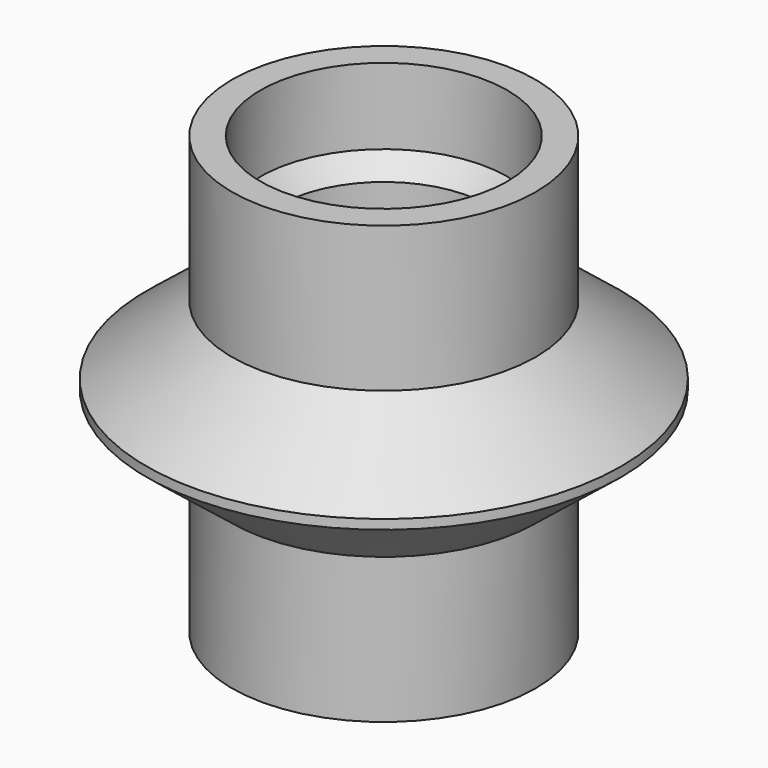
from build123d import *

# Parameters (mm, degrees)
F0_R         = 8
F0_R_2       = 6.5
F1_DEPTH     = 11.5
F0_R_3       = 12.5
F2_DEPTH     = 4.25
F3_S5_R      = 8
F3_T6_DEPTH  = 19
F3_S11_R     = 8
F3_T12_DEPTH = 19
F0_R_4       = 5.5
F5_DEPTH     = 7.5
F6_SIZE      = 0.99999


# Not quite as in the source:
# - a fillet or chamfer that OpenCascade refuses, or shapes differently, is made with other operations: its cross-section is extruded or revolved along the edge and cut away or added
# - two fillets or chamfers of one size are made in one step
# - a fillet or chamfer is up to 0.001 mm smaller than in the source, because OpenCascade refuses the exact size


with BuildPart() as f1:
    # F0 (on Top) → F1 (new body, symmetric)
    with BuildSketch(Plane.XY):
        Circle(F0_R)
        Circle(F0_R_2, mode=Mode.SUBTRACT)
    extrude(amount=F1_DEPTH, both=True)

    # F0 (on Top) → F2 (join, symmetric)
    with BuildSketch(Plane.XY):
        Circle(F0_R_3)
        Circle(F0_R, mode=Mode.SUBTRACT)
    extrude(amount=F2_DEPTH, both=True)

    # F3: chamfer of 5 x 4 on 2 edges, made by hand


with BuildPart() as f3_tool2:
    # F3_s3 → F3_t4 (revolve)
    with BuildSketch(Plane.XZ):
        Polygon((12.5, 0.25), (7.5, 4.25), (12.5, 4.25), align=None)
    revolve(axis=Axis((0, 0, 4.25), (0, 0, 1)))

    # F3_s5 → F3_t6 (cut, symmetric)
    with BuildSketch(Plane.XY.offset(2.2)):
        Circle(F3_S5_R)
    extrude(amount=F3_T6_DEPTH, both=True, mode=Mode.SUBTRACT)


with BuildPart() as f1_1:
    add(f1.part)

    # F3_t1: cut F3_tool2
    add(f3_tool2.part, mode=Mode.SUBTRACT)


with BuildPart() as f3_tool8:
    # F3_s9 → F3_t10 (revolve)
    with BuildSketch(Plane.XZ):
        Polygon((7.5, -4.25), (12.5, -0.25), (12.5, -4.25), align=None)
    revolve(axis=Axis((0, 0, -4.25), (0, 0, 1)))

    # F3_s11 → F3_t12 (cut, symmetric)
    with BuildSketch(Plane.XY.offset(-2.2)):
        Circle(F3_S11_R)
    extrude(amount=F3_T12_DEPTH, both=True, mode=Mode.SUBTRACT)


with BuildPart() as f1_2:
    add(f1_1.part)

    # F3_t7: cut F3_tool8
    add(f3_tool8.part, mode=Mode.SUBTRACT)

    # F0 (on Top) → F5 (join, symmetric)
    with BuildSketch(Plane.XY):
        Circle(F0_R_2)
        Circle(F0_R_4, mode=Mode.SUBTRACT)
    extrude(amount=F5_DEPTH, both=True)

    # F6 (size 1 in the source; OpenCascade refuses exactly that, so slightly less here)
    f6_edges = [f1_2.edges().sort_by_distance(p)[0] for p in [
        (-5.5, 0, 7.5),
    ]]
    chamfer(f6_edges, length=F6_SIZE)


solid = f1_2.part
